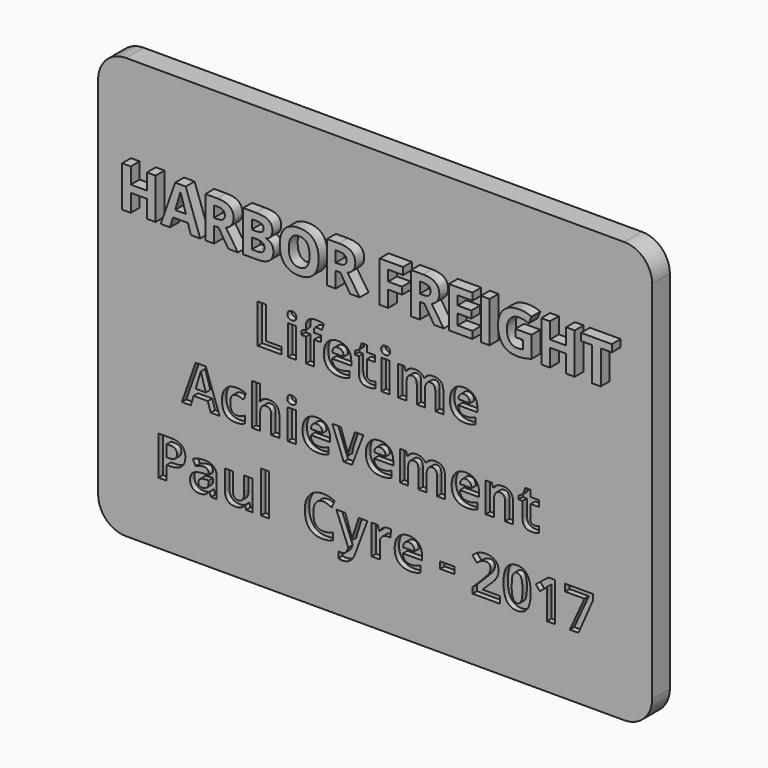
from build123d import *

# Parameters (mm, degrees)
F0_W         = 100
F0_H         = 76
F1_DEPTH     = 4
F2_TEXT_SIZE = 10.3253562786
F3_DEPTH     = 6
F4_TEXT_SIZE = 9.8489949024
F5_DEPTH     = 1
F6_R         = 5


# Not quite as in the source:
# - Text() gives the source's letters only with a copy of the font that has no kerning and outlines rounded to 1/6400 em; it was checked with that copy


with BuildPart() as f1:
    # F0 (on Front) → F1 (new body)
    with BuildSketch(Plane.XZ):
        Rectangle(F0_W, F0_H)
    extrude(amount=F1_DEPTH)

    # F2 (on Front) → F3 (join)
    with BuildSketch(Plane.XZ):
        with Locations((-45, 15)):
            Text('HARBOR FREIGHT', F2_TEXT_SIZE, font='Open Sans', font_style=FontStyle.BOLD, text_align=(TextAlign.LEFT, TextAlign.BOTTOM))
    extrude(amount=F3_DEPTH)

    # F4 (on face) → F5 (cut)
    with BuildSketch(Plane.XZ.offset(4)):
        with Locations((-22.0856016159, 0)):
            Text('Lifetime', F4_TEXT_SIZE, font='Open Sans', font_style=FontStyle.BOLD, text_align=(TextAlign.LEFT, TextAlign.BOTTOM))
        with Locations((-34.8816004617, -13.3946330672)):
            Text('Achievement', F4_TEXT_SIZE, font='Open Sans', font_style=FontStyle.BOLD, text_align=(TextAlign.LEFT, TextAlign.BOTTOM))
        with Locations((-40, -26.7892661345)):
            Text('Paul  Cyre - 2017', F4_TEXT_SIZE, font='Open Sans', font_style=FontStyle.BOLD, text_align=(TextAlign.LEFT, TextAlign.BOTTOM))
    extrude(amount=-F5_DEPTH, mode=Mode.SUBTRACT)

    # F6
    f6_edges = [f1.edges().sort_by_distance(p)[0] for p in [
        (-50, -2, 38),
        (-50, -2, -38),
        (50, -2, -38),
        (50, -2, 38),
    ]]
    fillet(f6_edges, radius=F6_R)


solid = f1.part
